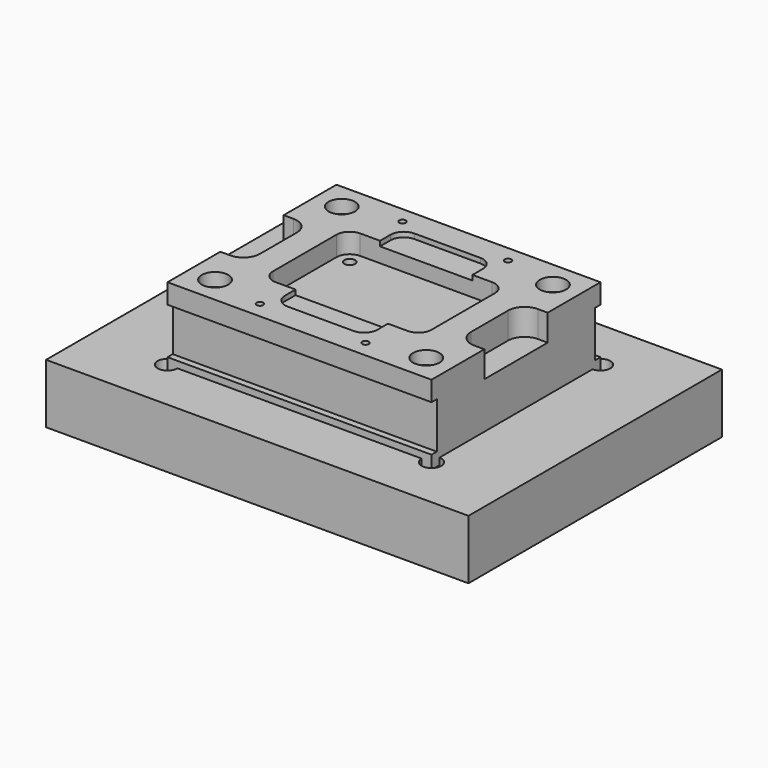
from build123d import *

# Parameters (mm, degrees)
F0_W           = 127
F0_H           = 101.6
F1_DEPTH       = 38.1
F2_W           = 76.2
F2_H           = 50.8
F3_DEPTH       = 9.525
F4_R           = 6.35
F6_D           = 6.35
F6_CBORE_D     = 12.7
F6_CBORE_DEPTH = 6.35
F7_W           = 3.175
F7_H           = 22.225
F8_DEPTH       = 127.001
F10_D          = 5.1054
F10_DEPTH      = 19.05
F10_TIP        = 1.5338169022
F11_W          = 12.7
F11_H          = 38.1
F12_DEPTH      = 12.7
F13_R          = 7.9375
F15_DEPTH      = 3.175
F16_W          = 57.15
F16_H          = 31.75
F17_DEPTH      = 6.35
F18_R          = 6.35
F20_D          = 3.175
F20_DEPTH      = 9.525
F20_TIP        = 0.9538662327
F21_W          = 44.45
F21_H          = 76.2
F22_DEPTH      = 2.38125
F23_R          = 6.35
F24_W          = 203.2
F24_H          = 152.4
F25_DEPTH      = 25.4
F25_DEPTH_BACK = 3.175
F26_W          = 127
F26_H          = 101.6
F27_DEPTH      = 3.175
F28_R          = 4.7625
F29_DEPTH      = 28.576


with BuildPart() as f1:
    # F0 (on Top) → F1 (new body)
    with BuildSketch(Plane.XY):
        Rectangle(F0_W, F0_H)
    extrude(amount=F1_DEPTH)

    # F2 (on face) → F3 (cut)
    with BuildSketch(Plane.XY.offset(38.1)):
        Rectangle(F2_W, F2_H)
    extrude(amount=-F3_DEPTH, mode=Mode.SUBTRACT)

    # F4
    f4_edges = [f1.edges().sort_by_distance(p)[0] for p in [
        (-38.1, 25.4, 33.3375),
        (38.1, 25.4, 33.3375),
        (38.1, -25.4, 33.3375),
        (-38.1, -25.4, 33.3375),
    ]]
    fillet(f4_edges, radius=F4_R)

    # F6 (through all)
    with Locations(Plane.XY.offset(38.1)):
        with Locations((-50.8, 38.1), (50.8, 38.1), (50.8, -38.1), (-50.8, -38.1)):
            CounterBoreHole(F6_D / 2, F6_CBORE_D / 2, F6_CBORE_DEPTH)

    # F7 (on face) → F8 (cut, through all)
    with BuildSketch(Plane.YZ.offset(63.5)):
        with Locations((-49.2125, 17.4625)):
            Rectangle(F7_W, F7_H)
        with Locations((49.2125, 17.4625)):
            Rectangle(F7_W, F7_H)
    extrude(amount=-F8_DEPTH, mode=Mode.SUBTRACT)

    # F10
    with Locations(Plane.XY.offset(28.575)):
        with Locations((-31.75, 19.05), (-31.75, -19.05), (31.75, -19.05), (31.75, 19.05)):
            Hole(F10_D / 2, depth=F10_DEPTH)
            with Locations((0, 0, -(F10_DEPTH + F10_TIP / 2))):  # 118° drill point
                Cone(0, F10_D / 2, F10_TIP, mode=Mode.SUBTRACT)

    # F11 (on face) → F12 (cut)
    with BuildSketch(Plane.XY.offset(38.1)):
        with Locations((-57.15, 0)):
            Rectangle(F11_W, F11_H)
        with Locations((57.15, 0)):
            Rectangle(F11_W, F11_H)
    extrude(amount=-F12_DEPTH, mode=Mode.SUBTRACT)

    # F13
    f13_edges = [f1.edges().sort_by_distance(p)[0] for p in [
        (-50.8, 19.05, 31.75),
        (-50.8, -19.05, 31.75),
        (50.8, 19.05, 31.75),
        (50.8, -19.05, 31.75),
    ]]
    fillet(f13_edges, radius=F13_R)

    # F14 (on face) → F15 (cut)
    with BuildSketch(Plane(origin=(0, 0, 0), x_dir=(1, 0, 0), z_dir=(0, 0, -1))):
        with BuildLine():
            Line((-31.75, -25.4), (31.75, -25.4))
            ThreePointArc((31.75, -25.4), (36.2401280605, -23.5401280605), (38.1, -19.05))
            Line((38.1, -19.05), (38.1, 19.05))
            ThreePointArc((38.1, 19.05), (36.2401280605, 23.5401280605), (31.75, 25.4))
            Line((31.75, 25.4), (-31.75, 25.4))
            ThreePointArc((-31.75, 25.4), (-36.2401280605, 23.5401280605), (-38.1, 19.05))
            Line((-38.1, 19.05), (-38.1, -19.05))
            ThreePointArc((-38.1, -19.05), (-36.2401280605, -23.5401280605), (-31.75, -25.4))
        make_face()
    extrude(amount=-F15_DEPTH, mode=Mode.SUBTRACT)

    # F16 (on face) → F17 (cut)
    with BuildSketch(Plane(origin=(0, 0, 3.175), x_dir=(1, 0, 0), z_dir=(0, 0, -1))):
        Rectangle(F16_W, F16_H)
    extrude(amount=-F17_DEPTH, mode=Mode.SUBTRACT)

    # F18
    f18_edges = [f1.edges().sort_by_distance(p)[0] for p in [
        (-28.575, -15.875, 6.35),
        (-28.575, 15.875, 6.35),
        (28.575, -15.875, 6.35),
        (28.575, 15.875, 6.35),
    ]]
    fillet(f18_edges, radius=F18_R)

    # F20
    with Locations(Plane.XY.offset(38.1)):
        with Locations((-25.4, 42.8625), (25.4, 42.8625), (-25.4, -42.8625), (25.4, -42.8625)):
            Hole(F20_D / 2, depth=F20_DEPTH)
            with Locations((0, 0, -(F20_DEPTH + F20_TIP / 2))):  # 118° drill point
                Cone(0, F20_D / 2, F20_TIP, mode=Mode.SUBTRACT)

    # F21 (on face) → F22 (cut)
    with BuildSketch(Plane.XY.offset(38.1)):
        Rectangle(F21_W, F21_H)
    extrude(amount=-F22_DEPTH, mode=Mode.SUBTRACT)

    # F23
    f23_edges = [f1.edges().sort_by_distance(p)[0] for p in [
        (-22.225, 38.1, 36.909375),
        (22.225, 38.1, 36.909375),
        (22.225, -38.1, 36.909375),
        (-22.225, -38.1, 36.909375),
    ]]
    fillet(f23_edges, radius=F23_R)


with BuildPart() as f25:
    # F24 (on face) → F25 (new body, two sides)
    with BuildSketch(Plane(origin=(0, 0, 0), x_dir=(1, 0, 0), z_dir=(0, 0, -1))) as f25_sk:
        Rectangle(F24_W, F24_H)
    extrude(amount=F25_DEPTH)
    extrude(f25_sk.sketch, amount=-F25_DEPTH_BACK)

    # F26 (on face) → F27 (cut)
    with BuildSketch(Plane.XY.offset(3.175)):
        Rectangle(F26_W, F26_H)
    extrude(amount=-F27_DEPTH, mode=Mode.SUBTRACT)

    # F28 (on face) → F29 (cut, through all)
    with BuildSketch(Plane.XY.offset(3.175)):
        with Locations((-63.5, 50.8)):
            Circle(F28_R)
        with Locations((-63.5, -50.8)):
            Circle(F28_R)
        with Locations((63.5, 50.8)):
            Circle(F28_R)
        with Locations((63.5, -50.8)):
            Circle(F28_R)
    extrude(amount=-F29_DEPTH, mode=Mode.SUBTRACT)


solid = Compound([f1.part, f25.part])
